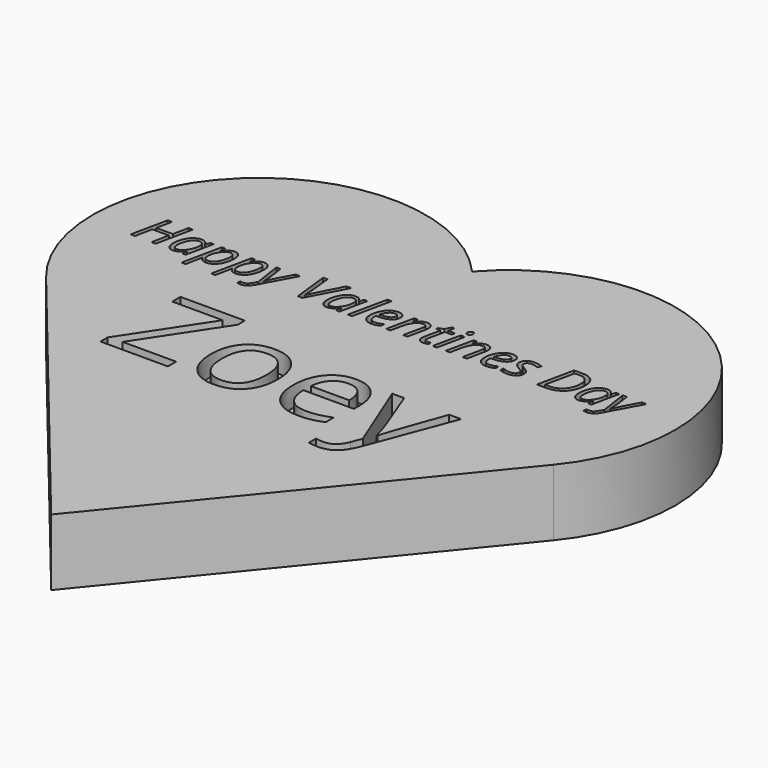
from build123d import *

# Parameters (mm, degrees)
F1_DEPTH       = 5.08
F2_TEXT_SIZE   = 3.928784339
F2_TEXT_SIZE_2 = 10.4766395251
F3_DEPTH       = 1.524


# Not quite as in the source:
# - Text() gives the source's letters only with a copy of the font that has no kerning and outlines rounded to 1/6400 em; it was checked with that copy


with BuildPart() as f1:
    # F0 (on Top) → F1 (new body)
    with BuildSketch(Plane.XY):
        with BuildLine():
            ThreePointArc((19.3630151068, -3.4200347289), (17.742323033, 14.2946338278), (0, 13.0116302157))
            ThreePointArc((0, 13.0116302157), (-17.742323033, 14.2946338278), (-19.3630151068, -3.4200347289))
            Line((-19.3630151068, -3.4200347289), (0, -27.1386301969))
            Line((0, -27.1386301969), (19.3630151068, -3.4200347289))
        make_face()
    extrude(amount=F1_DEPTH)

    # F2 (on face) → F3 (cut)
    with BuildSketch(Plane.XY.offset(5.08)):
        with Locations((-19.05, 4.0428909249)):
            Text('Happy Valentines Day', F2_TEXT_SIZE, font='Open Sans', font_style=FontStyle.ITALIC, text_align=(TextAlign.LEFT, TextAlign.BOTTOM))
        with Locations((-12.067779153, -7.873645719)):
            Text('Zoey', F2_TEXT_SIZE_2, font='Open Sans', text_align=(TextAlign.LEFT, TextAlign.BOTTOM))
    extrude(amount=-F3_DEPTH, mode=Mode.SUBTRACT)


solid = f1.part
